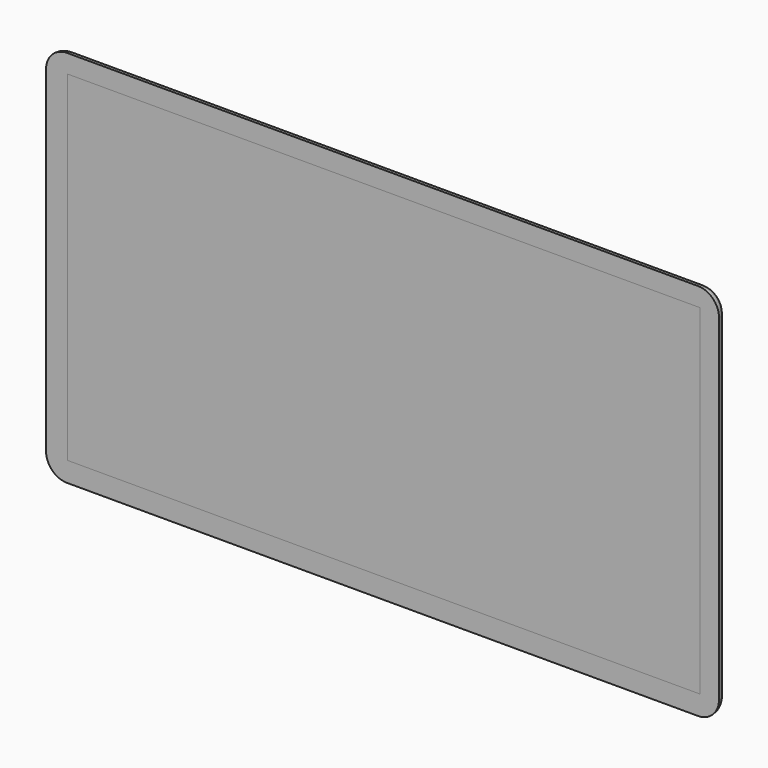
from build123d import *

# Parameters (mm, degrees)
F0_W         = 1600
F0_H         = 900
F0_W_2       = 1504.2692422867
F0_H_2       = 808.7469339371
F1_DEPTH     = 25
F2_W         = 1504.2692422867
F2_H         = 808.7469339371
F3_DEPTH     = 15
F4_R         = 50
F5_T1_DEPTH  = 808.7469339371
F5_T3_DEPTH  = 1504.2692422867
F5_T5_DEPTH  = 800
F5_T7_DEPTH  = 1500
F5_T10_ANGLE = 90
F5_T12_ANGLE = 90
F5_T14_ANGLE = 90
F5_T16_ANGLE = 90
F5_T21_DEPTH = 1566.7692422867
F5_T25_DEPTH = 871.2469339371
F5_T32_DEPTH = 871.2469339371
F5_T36_DEPTH = 1566.7692422867
F5_T43_DEPTH = 1566.7692422867
F5_T47_DEPTH = 871.2469339371
F5_T54_DEPTH = 1566.7692422867
F5_T58_DEPTH = 871.2469339371


# Not quite as in the source:
# - a fillet or chamfer that OpenCascade refuses, or shapes differently, is made with other operations: its cross-section is extruded or revolved along the edge and cut away or added


with BuildPart() as f1:
    # F0 (on Front) → F1 (new body)
    with BuildSketch(Plane.XZ):
        with Locations((1.7499998212, -58.5693205115)):
            Rectangle(F0_W, F0_H)
        with Locations((4.9877166748, -56.7320287228)):
            Rectangle(F0_W_2, F0_H_2, mode=Mode.SUBTRACT)
    extrude(amount=F1_DEPTH)

    # F4
    f4_edges = [f1.edges().sort_by_distance(p)[0] for p in [
        (801.75, -12.5, 391.430679),
        (801.75, -12.5, -508.569321),
        (-798.25, -12.5, -508.569321),
        (-798.25, -12.5, 391.430679),
    ]]
    fillet(f4_edges, radius=F4_R)

    # F5: fillet of radius 25 on 12 edges, made by hand

    # F5_s2 → F5_t1 (cut)
    with BuildSketch(Plane.XY.offset(-461.1054956913)):
        with BuildLine():
            ThreePointArc((782.1223378181, 0), (764.4446682885, -7.3223304703), (757.1223378181, -25))
            Line((757.1223378181, -25), (757.1223378181, 0))
            Line((757.1223378181, 0), (782.1223378181, 0))
        make_face()
        with BuildLine():
            ThreePointArc((-772.1469044685, 0), (-754.4692349389, -7.3223304703), (-747.1469044685, -25))
            Line((-747.1469044685, -25), (-747.1469044685, 0))
            Line((-747.1469044685, 0), (-772.1469044685, 0))
        make_face()
    extrude(amount=F5_T1_DEPTH, mode=Mode.SUBTRACT)

    # F5_s4 → F5_t3 (cut)
    with BuildSketch(Plane.YZ.offset(-747.1469044685)):
        with BuildLine():
            ThreePointArc((0, 372.6414382458), (-7.3223304703, 354.9637687161), (-25, 347.6414382458))
            Line((-25, 347.6414382458), (0, 347.6414382458))
            Line((0, 347.6414382458), (0, 372.6414382458))
        make_face()
        with BuildLine():
            ThreePointArc((0, -486.1054956913), (-7.3223304703, -468.4278261616), (-25, -461.1054956913))
            Line((-25, -461.1054956913), (0, -461.1054956913))
            Line((0, -461.1054956913), (0, -486.1054956913))
        make_face()
    extrude(amount=F5_T3_DEPTH, mode=Mode.SUBTRACT)

    # F5_s6 → F5_t5 (cut)
    with BuildSketch(Plane.XY.offset(-458.5693205115)):
        with BuildLine():
            ThreePointArc((-773.2500001788, 0), (-790.9276697085, -7.3223304703), (-798.2500001788, -25))
            Line((-798.2500001788, -25), (-798.2500001788, 0))
            Line((-798.2500001788, 0), (-773.2500001788, 0))
        make_face()
        with BuildLine():
            ThreePointArc((801.7499998212, -25), (794.4276693508, -7.3223304703), (776.7499998212, 0))
            Line((776.7499998212, 0), (801.7499998212, 0))
            Line((801.7499998212, 0), (801.7499998212, -25))
        make_face()
    extrude(amount=F5_T5_DEPTH, mode=Mode.SUBTRACT)

    # F5_s8 → F5_t7 (cut)
    with BuildSketch(Plane.YZ.offset(-748.2500001788)):
        with BuildLine():
            ThreePointArc((0, 366.4306794885), (-7.3223304703, 384.1083490182), (-25, 391.4306794885))
            Line((-25, 391.4306794885), (0, 391.4306794885))
            Line((0, 391.4306794885), (0, 366.4306794885))
        make_face()
        with BuildLine():
            ThreePointArc((0, -483.5693205115), (-7.3223304703, -501.2469900411), (-25, -508.5693205115))
            Line((-25, -508.5693205115), (0, -508.5693205115))
            Line((0, -508.5693205115), (0, -483.5693205115))
        make_face()
    extrude(amount=F5_T7_DEPTH, mode=Mode.SUBTRACT)

    # F5_s9 → F5_t10 (revolve, cut)
    with BuildSketch(Plane.YZ.offset(-748.2500001788)):
        with BuildLine():
            ThreePointArc((0, 366.4306794885), (-7.3223304703, 384.1083490182), (-25, 391.4306794885))
            Line((-25, 391.4306794885), (0, 391.4306794885))
            Line((0, 391.4306794885), (0, 366.4306794885))
        make_face()
    revolve(axis=Axis((-748.2500001788, 0, 341.4306794885), (0, -1, 0)), revolution_arc=F5_T10_ANGLE, mode=Mode.SUBTRACT)

    # F5_s11 → F5_t12 (revolve, cut)
    with BuildSketch(Plane.XY.offset(341.4306794885)):
        with BuildLine():
            ThreePointArc((776.7499998212, 0), (794.4276693508, -7.3223304703), (801.7499998212, -25))
            Line((801.7499998212, -25), (801.7499998212, 0))
            Line((801.7499998212, 0), (776.7499998212, 0))
        make_face()
    revolve(axis=Axis((751.7499998212, 0, 341.4306794885), (0, -1, 0)), revolution_arc=F5_T12_ANGLE, mode=Mode.SUBTRACT)

    # F5_s13 → F5_t14 (revolve, cut)
    with BuildSketch(Plane.XY.offset(-458.5693205115)):
        with BuildLine():
            ThreePointArc((776.7499998212, 0), (794.4276693508, -7.3223304703), (801.7499998212, -25))
            Line((801.7499998212, -25), (801.7499998212, 0))
            Line((801.7499998212, 0), (776.7499998212, 0))
        make_face()
    revolve(axis=Axis((751.7499998212, 0, -458.5693205115), (0, 1, 0)), revolution_arc=F5_T14_ANGLE, mode=Mode.SUBTRACT)

    # F5_s15 → F5_t16 (revolve, cut)
    with BuildSketch(Plane.XY.offset(-458.5693205115)):
        with BuildLine():
            ThreePointArc((-773.2500001788, 0), (-790.9276697085, -7.3223304703), (-798.2500001788, -25))
            Line((-798.2500001788, -25), (-798.2500001788, 0))
            Line((-798.2500001788, 0), (-773.2500001788, 0))
        make_face()
    revolve(axis=Axis((-748.2500001788, 0, -458.5693205115), (0, -1, 0)), revolution_arc=F5_T16_ANGLE, mode=Mode.SUBTRACT)


with BuildPart() as f3:
    # F2 (on face) → F3 (new body)
    with BuildSketch(Plane.XZ.offset(25)):
        with Locations((4.9877166748, -56.7320287228)):
            Rectangle(F2_W, F2_H)
    extrude(amount=-F3_DEPTH)


with BuildPart() as f5_tool19:
    # F5_s20 → F5_t21 (new body)
    with BuildSketch(Plane.YZ.offset(-747.1469044685)):
        with BuildLine():
            ThreePointArc((0, 372.6414382458), (-7.3223304703, 354.9637687161), (-25, 347.6414382458))
            Line((-25, 347.6414382458), (0, 347.6414382458))
            Line((0, 347.6414382458), (0, 372.6414382458))
        make_face()
    extrude(amount=F5_T21_DEPTH)

    split(bisect_by=Plane.YZ.offset(757.1223378181), keep=Keep.TOP)


with BuildPart() as f5_tool23:
    # F5_s24 → F5_t25 (new body)
    with BuildSketch(Plane.XY.offset(410.1414382458)):
        with BuildLine():
            ThreePointArc((782.1223378181, 0), (764.4446682885, -7.3223304703), (757.1223378181, -25))
            Line((757.1223378181, -25), (757.1223378181, 0))
            Line((757.1223378181, 0), (782.1223378181, 0))
        make_face()
    extrude(amount=-F5_T25_DEPTH)

    split(bisect_by=Plane.XY.offset(347.6414382458), keep=Keep.TOP)


with BuildPart() as f5_tool19_1:
    add(f5_tool19.part)

    # F5_t27: intersect F5_tool23
    add(f5_tool23.part, mode=Mode.INTERSECT)


with BuildPart() as f1_1:
    add(f1.part)

    # F5_t17: cut F5_tool19
    add(f5_tool19_1.part, mode=Mode.SUBTRACT)


with BuildPart() as f5_tool30:
    # F5_s31 → F5_t32 (new body)
    with BuildSketch(Plane.XY.offset(347.6414382458)):
        with BuildLine():
            ThreePointArc((782.1223378181, 0), (764.4446682885, -7.3223304703), (757.1223378181, -25))
            Line((757.1223378181, -25), (757.1223378181, 0))
            Line((757.1223378181, 0), (782.1223378181, 0))
        make_face()
    extrude(amount=-F5_T32_DEPTH)

    split(bisect_by=Plane.XY.offset(-461.1054956913), keep=Keep.BOTTOM)


with BuildPart() as f5_tool34:
    # F5_s35 → F5_t36 (new body)
    with BuildSketch(Plane.YZ.offset(819.6223378181)):
        with BuildLine():
            ThreePointArc((0, -486.1054956913), (-7.3223304703, -468.4278261616), (-25, -461.1054956913))
            Line((-25, -461.1054956913), (0, -461.1054956913))
            Line((0, -461.1054956913), (0, -486.1054956913))
        make_face()
    extrude(amount=-F5_T36_DEPTH)

    split(bisect_by=Plane.YZ.offset(757.1223378181), keep=Keep.TOP)


with BuildPart() as f5_tool30_1:
    add(f5_tool30.part)

    # F5_t38: intersect F5_tool34
    add(f5_tool34.part, mode=Mode.INTERSECT)


with BuildPart() as f1_2:
    add(f1_1.part)

    # F5_t28: cut F5_tool30
    add(f5_tool30_1.part, mode=Mode.SUBTRACT)


with BuildPart() as f5_tool41:
    # F5_s42 → F5_t43 (new body)
    with BuildSketch(Plane.YZ.offset(-809.6469044685)):
        with BuildLine():
            ThreePointArc((0, 372.6414382458), (-7.3223304703, 354.9637687161), (-25, 347.6414382458))
            Line((-25, 347.6414382458), (0, 347.6414382458))
            Line((0, 347.6414382458), (0, 372.6414382458))
        make_face()
    extrude(amount=F5_T43_DEPTH)

    split(bisect_by=Plane.YZ.offset(-747.1469044685), keep=Keep.BOTTOM)


with BuildPart() as f5_tool45:
    # F5_s46 → F5_t47 (new body)
    with BuildSketch(Plane.XY.offset(-461.1054956913)):
        with BuildLine():
            ThreePointArc((-772.1469044685, 0), (-754.4692349389, -7.3223304703), (-747.1469044685, -25))
            Line((-747.1469044685, -25), (-747.1469044685, 0))
            Line((-747.1469044685, 0), (-772.1469044685, 0))
        make_face()
    extrude(amount=F5_T47_DEPTH)

    split(bisect_by=Plane.XY.offset(347.6414382458), keep=Keep.TOP)


with BuildPart() as f5_tool41_1:
    add(f5_tool41.part)

    # F5_t49: intersect F5_tool45
    add(f5_tool45.part, mode=Mode.INTERSECT)


with BuildPart() as f1_3:
    add(f1_2.part)

    # F5_t39: cut F5_tool41
    add(f5_tool41_1.part, mode=Mode.SUBTRACT)


with BuildPart() as f5_tool52:
    # F5_s53 → F5_t54 (new body)
    with BuildSketch(Plane.YZ.offset(757.1223378181)):
        with BuildLine():
            ThreePointArc((0, -486.1054956913), (-7.3223304703, -468.4278261616), (-25, -461.1054956913))
            Line((-25, -461.1054956913), (0, -461.1054956913))
            Line((0, -461.1054956913), (0, -486.1054956913))
        make_face()
    extrude(amount=-F5_T54_DEPTH)

    split(bisect_by=Plane.YZ.offset(-747.1469044685), keep=Keep.BOTTOM)


with BuildPart() as f5_tool56:
    # F5_s57 → F5_t58 (new body)
    with BuildSketch(Plane.XY.offset(-523.6054956913)):
        with BuildLine():
            ThreePointArc((-772.1469044685, 0), (-754.4692349389, -7.3223304703), (-747.1469044685, -25))
            Line((-747.1469044685, -25), (-747.1469044685, 0))
            Line((-747.1469044685, 0), (-772.1469044685, 0))
        make_face()
    extrude(amount=F5_T58_DEPTH)

    split(bisect_by=Plane.XY.offset(-461.1054956913), keep=Keep.BOTTOM)


with BuildPart() as f5_tool52_1:
    add(f5_tool52.part)

    # F5_t60: intersect F5_tool56
    add(f5_tool56.part, mode=Mode.INTERSECT)


with BuildPart() as f1_4:
    add(f1_3.part)

    # F5_t50: cut F5_tool52
    add(f5_tool52_1.part, mode=Mode.SUBTRACT)


solid = Compound([f3.part, f1_4.part])
